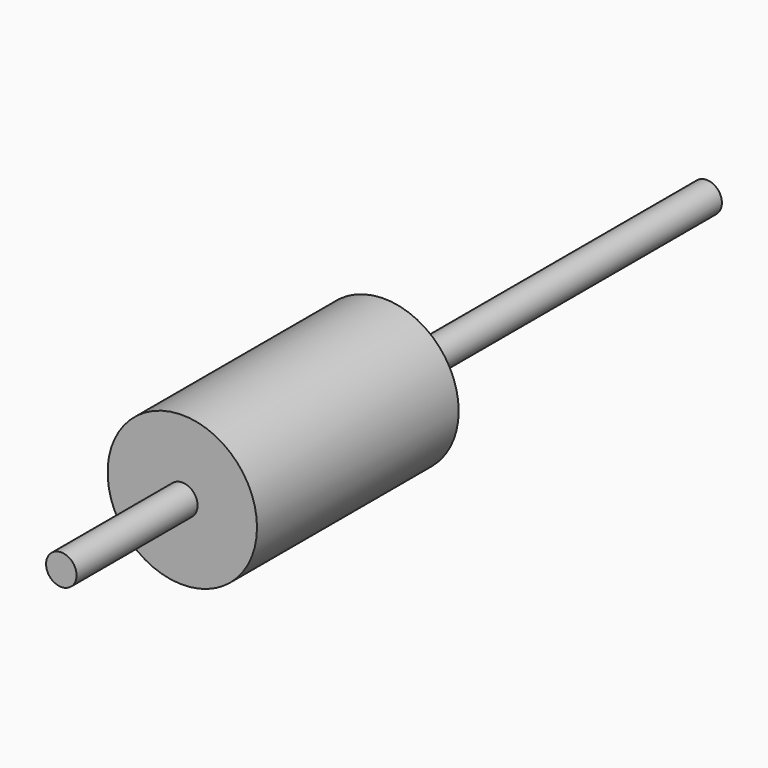
from build123d import *

# Parameters (mm, degrees)
F1_R     = 3.8443806978
F2_DEPTH = 101.6
F4_R     = 18.816397341
F5_DEPTH = 63.5


# Not quite as in the source:
# - the program builds the solid bodies; features that only make, move or delete a surface that nothing else refers to are left out


with BuildPart() as f2:
    # F1 (on Front) → F2 (new body, symmetric)
    with BuildSketch(Plane.XZ):
        Circle(F1_R)
    extrude(amount=F2_DEPTH, both=True)


with BuildPart() as f5:
    # F4 (on Front) → F5 (new body)
    with BuildSketch(Plane.XZ):
        Circle(F4_R)
    extrude(amount=F5_DEPTH)


solid = Compound([f2.part, f5.part])
